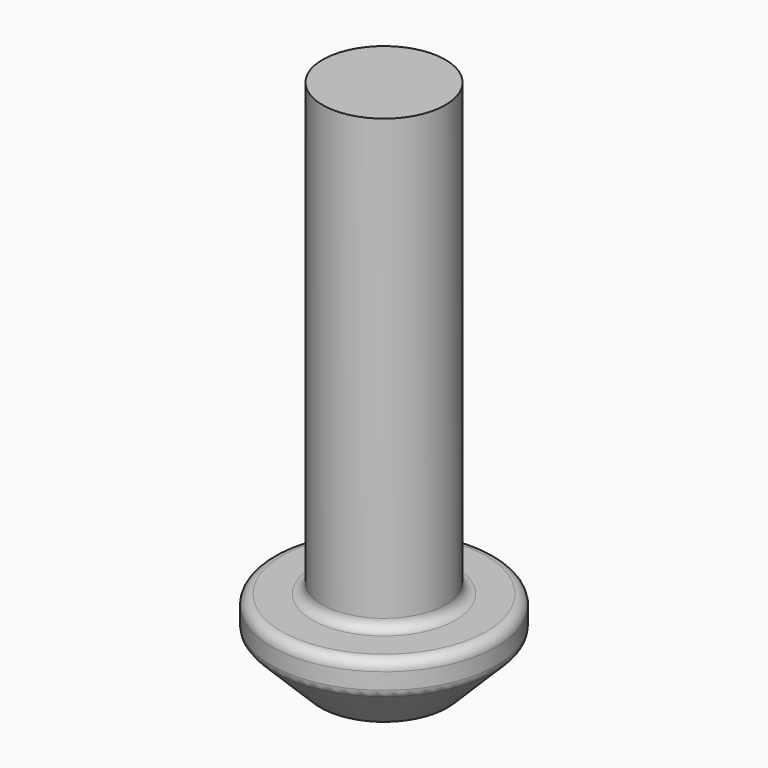
from build123d import *

# Parameters (mm, degrees)
F1_R     = 2.75
F1_R_2   = 1.5
F2_DEPTH = 2
F3_START = 1.5
F3_DEPTH = 0.5
F4_START = 2
F4_DEPTH = 11
F5_SIZE2 = 1.25
F5_SIZE  = 1.25
F6_R     = 0.25


# Not quite as in the source:
# - a feature names something its author has since deleted; it is built from what else it names


with BuildPart() as f2:
    # F1 (on Top) → F2 (new body)
    with BuildSketch(Plane.XY):
        Circle(F1_R)
        Circle(F1_R_2, mode=Mode.SUBTRACT)
        Circle(F1_R_2)
        Polygon((-0.5773502692, -1), (-1.1547005384, 0), (-0.5773502692, 1), (0.5773502692, 1), (1.1547005384, 0), (0.5773502692, -1), align=None, mode=Mode.SUBTRACT)
    extrude(amount=F2_DEPTH)

    # F1 (on Top) → F3 (join)
    with BuildSketch(Plane.XY.offset(F3_START)):
        Polygon((-0.5773502692, 1), (-1.1547005384, 0), (-0.5773502692, -1), (0.5773502692, -1), (1.1547005384, 0), (0.5773502692, 1), align=None)
    extrude(amount=F3_DEPTH)

    # F1 (on Top) → F4 (join)
    with BuildSketch(Plane.XY.offset(F4_START)):
        Circle(F1_R_2)
        Polygon((-0.5773502692, -1), (-1.1547005384, 0), (-0.5773502692, 1), (0.5773502692, 1), (1.1547005384, 0), (0.5773502692, -1), align=None, mode=Mode.SUBTRACT)
        Polygon((-0.5773502692, 1), (-1.1547005384, 0), (-0.5773502692, -1), (0.5773502692, -1), (1.1547005384, 0), (0.5773502692, 1), align=None)
    extrude(amount=F4_DEPTH)

    # F5
    f5_edges = [f2.edges().sort_by_distance(p)[0] for p in [
        (-2.75, 0, 0),
    ]]
    chamfer(f5_edges, length=F5_SIZE, length2=F5_SIZE2)

    # F6
    f6_edges = [f2.edges().sort_by_distance(p)[0] for p in [
        (-2.75, 0, 2),
        (-1.5, 0, 2),
        (-1.5, 0, 0),
        (-2.75, 0, 1.25),
    ]]
    fillet(f6_edges, radius=F6_R)


solid = f2.part
